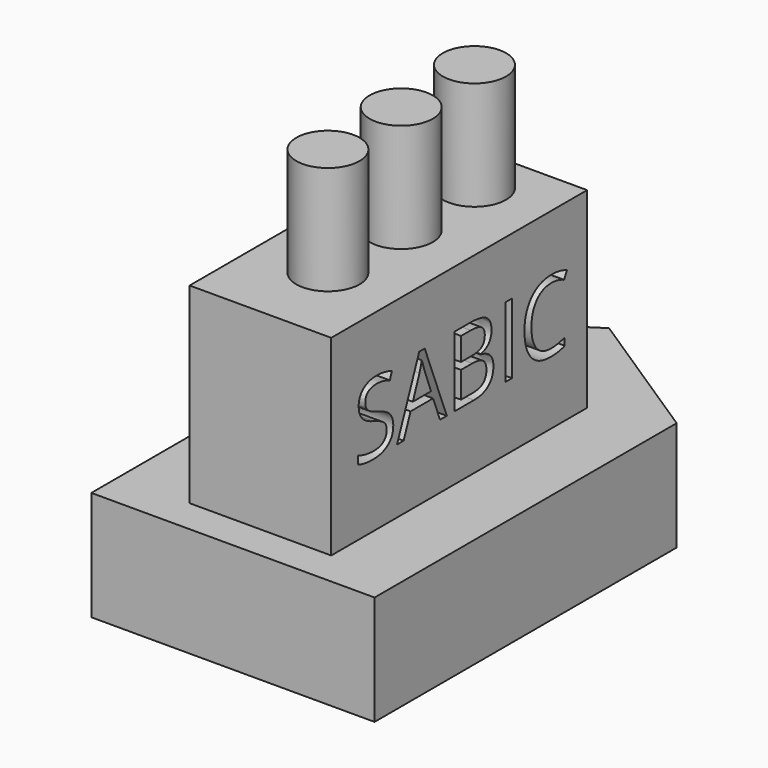
from build123d import *

# Parameters (mm, degrees)
F1_DEPTH     = 29.464
F2_W         = 38.1
F2_H         = 86.0539227724
F3_DEPTH     = 81.026
F4_R         = 8.509
F5_DEPTH     = 110.236
F6_TEXT_SIZE = 26.4398009542
F7_DEPTH     = 42.418


# Not quite as in the source:
# - Text() gives the source's letters only with a copy of the font that has no kerning and outlines rounded to 1/6400 em; it was checked with that copy


with BuildPart() as f1:
    # F0 (on Top) → F1 (new body)
    with BuildSketch(Plane.XY):
        Polygon((-38.1, 45.0133037895), (-38.1, -56.5809474811), (38.1, -56.5809474811), (38.1, 45.0133037895), (0, 69.9012022044), align=None)
    extrude(amount=F1_DEPTH)

    # F2 (on Top) → F3 (join)
    with BuildSketch(Plane.XY):
        with Locations((0, -4.31708619)):
            Rectangle(F2_W, F2_H)
    extrude(amount=F3_DEPTH)

    # F4 (on Top) → F5 (join)
    with BuildSketch(Plane.XY):
        with Locations((0, 24.638)):
            Circle(F4_R)
        Circle(F4_R)
        with Locations((0, -24.638)):
            Circle(F4_R)
    extrude(amount=F5_DEPTH)

    # F6 (on face) → F7 (cut)
    with BuildSketch(Plane.YZ.offset(19.05)):
        with Locations((-39.7240475762, 46.749343313)):
            Text('SABIC', F6_TEXT_SIZE, font='Open Sans', text_align=(TextAlign.LEFT, TextAlign.BOTTOM))
    extrude(amount=-F7_DEPTH, mode=Mode.SUBTRACT)


solid = f1.part
